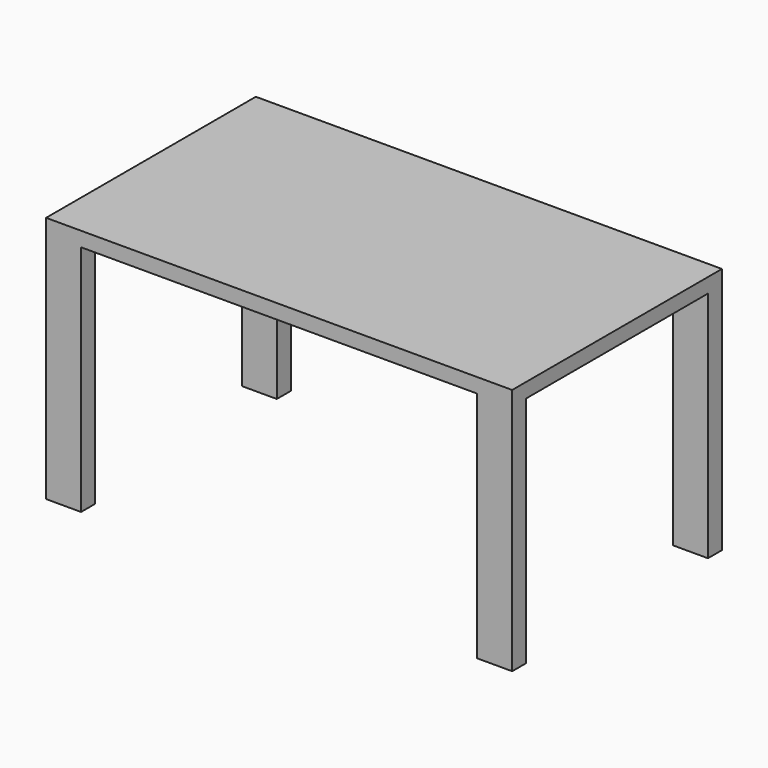
from build123d import *

# Parameters (mm, degrees)
F0_W     = 1600
F0_H     = 900
F1_DEPTH = 50
F2_W     = 120
F2_H     = 60
F3_DEPTH = 800


# Not quite as in the source:
# - a pattern or mirror of a feature is missing from the dataset's text; its kind, count and spacing are read off the source's solid


with BuildPart() as f1:
    # F0 (on Top) → F1 (new body)
    with BuildSketch(Plane.XY):
        Rectangle(F0_W, F0_H)
    extrude(amount=F1_DEPTH)

    # F2 (on face) → F3 (join)
    with BuildSketch(Plane(origin=(0, 0, 0), x_dir=(1, 0, 0), z_dir=(0, 0, -1))):
        with Locations((-740, 420)):
            Rectangle(F2_W, F2_H)
        with Locations((-740, -420)):
            Rectangle(F2_W, F2_H)
    f3 = extrude(amount=F3_DEPTH)

    # F3_copies: F3 across plane
    add(f3.mirror(Plane(origin=(0, 0, 0), x_dir=(0, 0, 1), z_dir=(1, 0, 0))))


solid = f1.part
